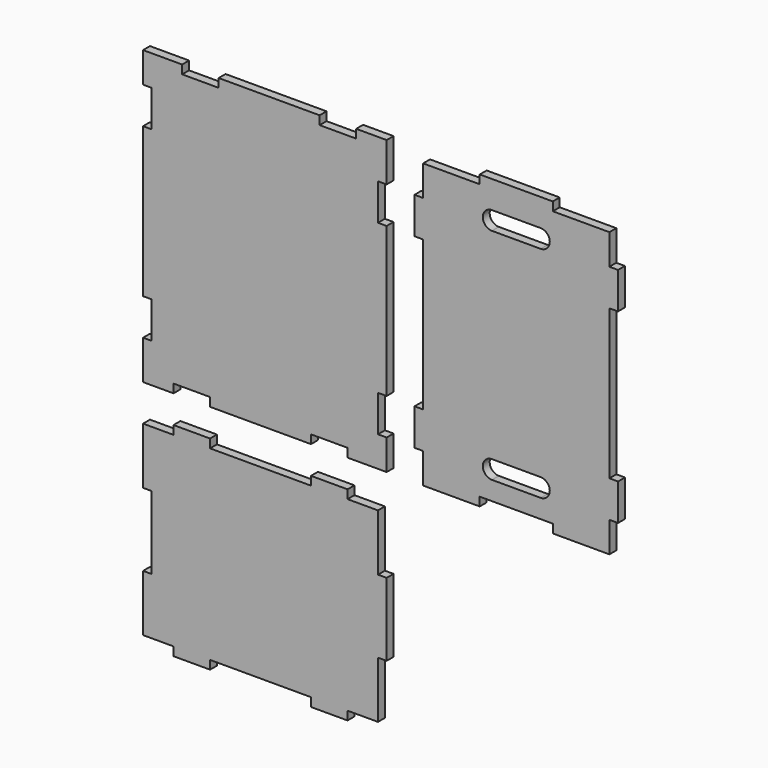
from build123d import *

# Parameters (mm, degrees)
F1_W     = 18.034
F1_H     = 152.4
F1_W_2   = 76.2
F1_H_2   = 18.034
F2_DEPTH = 18.034
F1_W_3   = 152.4
F1_H_3   = 76.2


# Not quite as in the source:
# - a variable given as a bare number and used for a length is read in inches; the dataset says mm whatever the document's units were
# - a feature names something its author has since deleted; it is built from what else it names


with BuildPart() as f2:
    # F1 (on Front) → F2 (new body)
    with BuildSketch(Plane.XZ):
        with Locations((254, 0)):
            Rectangle(F1_W, F1_H)
        with Locations((-143.383, 203.2)):
            Rectangle(F1_W_2, F1_H_2)
        with Locations((143.383, 203.2)):
            Rectangle(F1_W_2, F1_H_2)
        Polygon((-181.483, 194.183), (-244.983, 194.183), (-244.983, 76.2), (-226.949, 76.2), (-226.949, -76.2), (-244.983, -76.2), (-244.983, -194.183), (-181.483, -194.183), (-105.283, -194.183), (105.283, -194.183), (181.483, -194.183), (244.983, -194.183), (244.983, -76.2), (244.983, 76.2), (244.983, 194.183), (181.483, 194.183), (105.283, 194.183), (-105.283, 194.183), align=None)
        with Locations((-143.383, -203.2)):
            Rectangle(F1_W_2, F1_H_2)
        with Locations((143.383, -203.2)):
            Rectangle(F1_W_2, F1_H_2)
    extrude(amount=F2_DEPTH)


with BuildPart() as f2b:
    # F1 (on Front) → F2, piece 2 (new body)
    with BuildSketch(Plane.XZ):
        Polygon((-244.983, 351.917), (-244.983, 270.383), (-181.483, 270.383), (-181.483, 288.417), (-105.283, 288.417), (-105.283, 270.383), (105.283, 270.383), (105.283, 288.417), (181.483, 288.417), (181.483, 270.383), (263.017, 270.383), (263.017, 333.883), (244.983, 333.883), (244.983, 410.083), (263.017, 410.083), (263.017, 722.249), (244.983, 722.249), (244.983, 798.449), (263.017, 798.449), (263.017, 879.983), (199.517, 879.983), (199.517, 861.949), (123.317, 861.949), (123.317, 879.983), (-87.249, 879.983), (-87.249, 861.949), (-163.449, 861.949), (-163.449, 879.983), (-244.983, 879.983), (-244.983, 816.483), (-226.949, 816.483), (-226.949, 740.283), (-244.983, 740.283), (-244.983, 428.117), (-226.949, 428.117), (-226.949, 351.917), align=None)
    extrude(amount=F2_DEPTH)


with BuildPart() as f2c:
    # F1 (on Front) → F2, piece 3 (new body)
    with BuildSketch(Plane.XZ):
        Polygon((339.217, 333.883), (339.217, 270.383), (457.2, 270.383), (457.2, 288.417), (609.6, 288.417), (609.6, 270.383), (727.583, 270.383), (727.583, 333.883), (727.583, 410.083), (727.583, 722.249), (727.583, 798.449), (727.583, 861.949), (609.6, 861.949), (457.2, 861.949), (339.217, 861.949), (339.217, 798.449), (339.217, 722.249), (339.217, 410.083), align=None)
        with BuildLine():
            Line((533.4, 365.633), (584.2, 365.633))
            ThreePointArc((584.2, 365.633), (603.25, 346.583), (584.2, 327.533))
            Line((584.2, 327.533), (533.4, 327.533))
            Line((533.4, 327.533), (482.6, 327.533))
            ThreePointArc((482.6, 327.533), (463.55, 346.583), (482.6, 365.633))
            Line((482.6, 365.633), (533.4, 365.633))
        make_face(mode=Mode.SUBTRACT)
        with BuildLine():
            Line((482.6, 822.833), (533.4, 822.833))
            Line((533.4, 822.833), (584.2, 822.833))
            ThreePointArc((584.2, 822.833), (603.25, 803.783), (584.2, 784.733))
            Line((584.2, 784.733), (533.4, 784.733))
            Line((533.4, 784.733), (482.6, 784.733))
            ThreePointArc((482.6, 784.733), (463.55, 803.783), (482.6, 822.833))
        make_face(mode=Mode.SUBTRACT)
        with Locations((533.4, 870.966)):
            Rectangle(F1_W_3, F1_H_2)
        with Locations((330.2, 760.349)):
            Rectangle(F1_W, F1_H_3)
        with Locations((330.2, 371.983)):
            Rectangle(F1_W, F1_H_3)
        with Locations((736.6, 760.349)):
            Rectangle(F1_W, F1_H_3)
        with Locations((736.6, 371.983)):
            Rectangle(F1_W, F1_H_3)
    extrude(amount=F2_DEPTH)


solid = Compound([f2.part, f2b.part, f2c.part])
